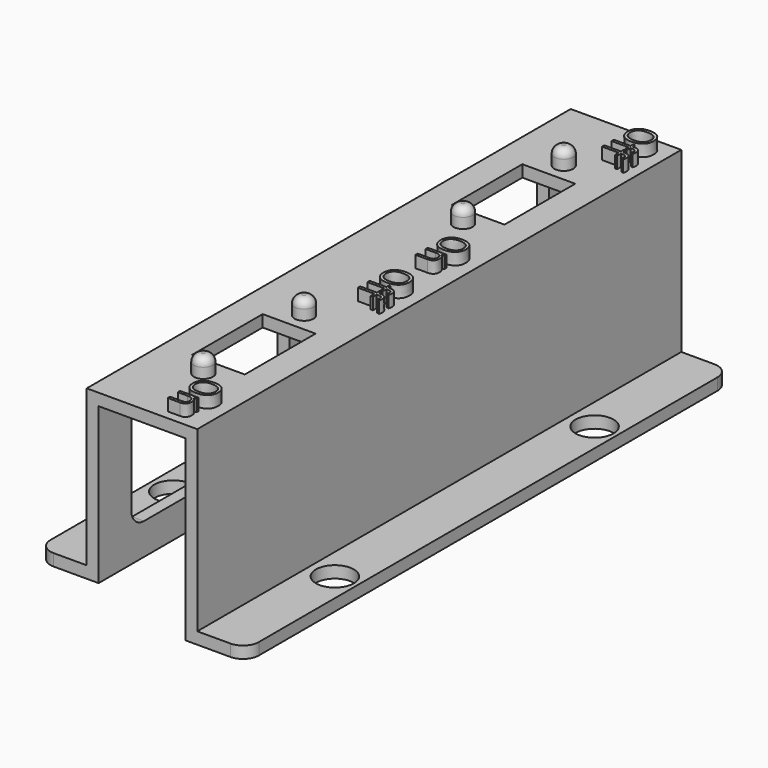
from build123d import *

# Parameters (mm, degrees)
F1_DEPTH        = 76.6
F2_R            = 2.4
F3_DEPTH        = 10
F4_W            = 25
F4_H            = 15
F5_DEPTH        = 1.5
F6_W            = 6.7
F6_H            = 11.2
F7_DEPTH        = 1.5
F8_R            = 1.2
F9_DEPTH        = 2.3
F10_R           = 1
F11_R           = 2
F12_R           = 2
F13_TEXT_SIZE   = 4.4746304435
F13_TEXT_SIZE_2 = 4.3576940536
F14_DEPTH       = 1.5


# Not quite as in the source:
# - Text() gives the source's letters only with a copy of the font that has no kerning and outlines rounded to 1/6400 em; it was checked with that copy


with BuildPart() as f1:
    # F0 (on Front) → F1 (new body)
    with BuildSketch(Plane.XZ):
        Polygon((0, 1.5), (0, 0), (7.69, 0), (7.69, 19.73), (18.69, 19.73), (18.69, -2.8), (26.38, -2.8), (26.38, -1.3), (20.19, -1.3), (20.19, 21.23), (6.19, 21.23), (6.19, 1.5), align=None)
    extrude(amount=F1_DEPTH)

    # F2 (on face) → F3 (cut)
    with BuildSketch(Plane.XY.offset(1.5)):
        with Locations((3, -17.82)):
            Circle(F2_R)
        with Locations((3, -58.92)):
            Circle(F2_R)
        with Locations((23.4651640058, -58.92)):
            Circle(F2_R)
        with Locations((23.4651640058, -17.82)):
            Circle(F2_R)
    extrude(amount=-F3_DEPTH, mode=Mode.SUBTRACT)

    # F4 (on face) → F5 (cut, through all)
    with BuildSketch(Plane(origin=(6.19, 0, 0), x_dir=(0, -1, 0), z_dir=(-1, 0, 0))):
        with Locations((17.82, 11.5)):
            Rectangle(F4_W, F4_H)
        with Locations((58.92, 11.5)):
            Rectangle(F4_W, F4_H)
    extrude(amount=-F5_DEPTH, mode=Mode.SUBTRACT)

    # F6 (on face) → F7 (cut, through all)
    with BuildSketch(Plane.XY.offset(21.23)):
        with Locations((13.19, -17.82)):
            Rectangle(F6_W, F6_H)
        with Locations((13.19, -58.92)):
            Rectangle(F6_W, F6_H)
    extrude(amount=-F7_DEPTH, mode=Mode.SUBTRACT)

    # F8 (on face) → F9 (join)
    with BuildSketch(Plane.XY.offset(21.23)):
        with Locations((13.19, -9.85)):
            Circle(F8_R)
        with Locations((13.19, -25.79)):
            Circle(F8_R)
        with Locations((13.19, -50.95)):
            Circle(F8_R)
        with Locations((13.19, -66.89)):
            Circle(F8_R)
    extrude(amount=F9_DEPTH)

    # F10
    f10_edges = [f1.edges().sort_by_distance(p)[0] for p in [
        (11.99, -9.85, 23.53),
        (11.99, -25.79, 23.53),
        (11.99, -50.95, 23.53),
        (11.99, -66.89, 23.53),
    ]]
    fillet(f10_edges, radius=F10_R)

    # F11
    f11_edges = [f1.edges().sort_by_distance(p)[0] for p in [
        (6.94, -5.32, 4),
        (6.94, -5.32, 19),
        (6.94, -30.32, 19),
        (6.94, -30.32, 4),
        (6.94, -46.42, 19),
        (6.94, -46.42, 4),
        (6.94, -71.42, 19),
        (6.94, -71.42, 4),
    ]]
    fillet(f11_edges, radius=F11_R)

    # F12
    f12_edges = [f1.edges().sort_by_distance(p)[0] for p in [
        (26.38, 0, -2.05),
        (0, 0, 0.75),
        (26.38, -76.6, -2.05),
        (0, -76.6, 0.75),
    ]]
    fillet(f12_edges, radius=F12_R)

    # F13 (on face) → F14 (join)
    with BuildSketch(Plane.XY.offset(21.23)):
        with Locations(Location((15.4580594707, -39.4219394555), (0, 0, -90))):
            Text('Off', F13_TEXT_SIZE, font='Open Sans', text_align=(TextAlign.LEFT, TextAlign.BOTTOM))
        with Locations(Location((15.5422536715, -69.7456515782), (0, 0, -90))):
            Text('On', F13_TEXT_SIZE_2, font='Open Sans', text_align=(TextAlign.LEFT, TextAlign.BOTTOM))
        with Locations(Location((15.4395983974, -0.7480261847), (0, 0, -90))):
            Text('Off', F13_TEXT_SIZE, font='Open Sans', text_align=(TextAlign.LEFT, TextAlign.BOTTOM))
        with Locations(Location((15.5237925981, -30.5067803711), (0, 0, -90))):
            Text('On', F13_TEXT_SIZE_2, font='Open Sans', text_align=(TextAlign.LEFT, TextAlign.BOTTOM))
    extrude(amount=F14_DEPTH)


solid = f1.part
